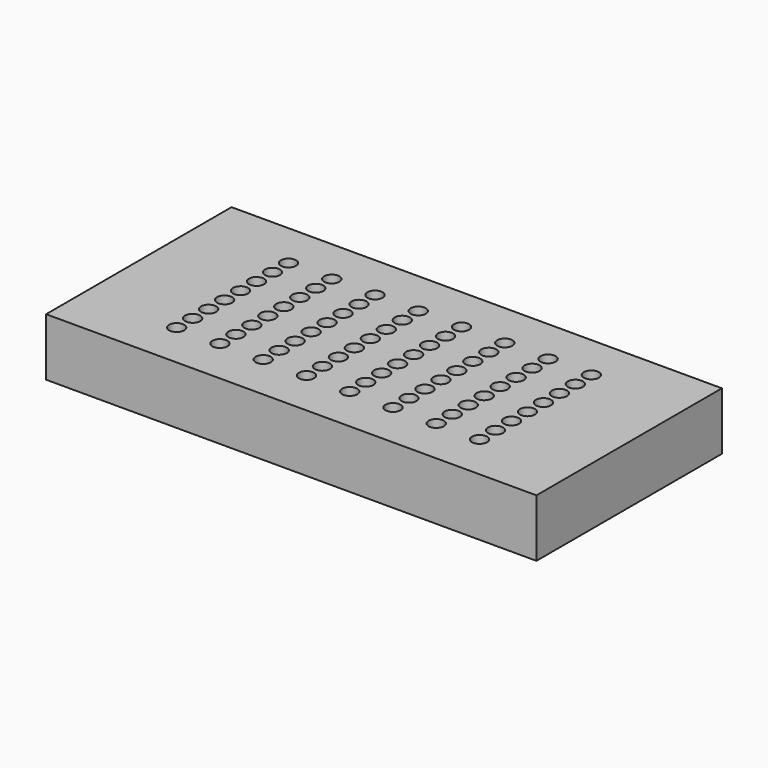
from build123d import *

# Parameters (mm, degrees)
F0_W     = 48
F0_H     = 22.15
F1_DEPTH = 4.98
F2_W     = 68
F2_H     = 32.15
F2_W_2   = 48
F2_H_2   = 22.15
F2_R     = 1.05
F3_DEPTH = 3
F4_DEPTH = 5


# Not quite as in the source:
# - a feature names something its author has since deleted; it is built from what else it names


with BuildPart() as f1:
    # F0 (on Top) → F1 (new body)
    with BuildSketch(Plane.XY):
        with Locations((-24, 11.075)):
            Rectangle(F0_W, F0_H)
    extrude(amount=F1_DEPTH)


with BuildPart() as f3:
    # F2 (on face) → F3 (new body)
    with BuildSketch(Plane.XY.offset(4.98)):
        with Locations((-24, 11.075)):
            Rectangle(F2_W, F2_H)
        with Locations((-24, 11.075)):
            Rectangle(F2_W_2, F2_H_2, mode=Mode.SUBTRACT)
        with Locations((-24, 11.075)):
            Rectangle(F2_W_2, F2_H_2)
        with Locations((-45, 1.384375)):
            Circle(F2_R, mode=Mode.SUBTRACT)
        with Locations((-39, 1.384375)):
            Circle(F2_R, mode=Mode.SUBTRACT)
        with Locations((-33, 1.384375)):
            Circle(F2_R, mode=Mode.SUBTRACT)
        with Locations((-27, 1.384375)):
            Circle(F2_R, mode=Mode.SUBTRACT)
        with Locations((-45, 4.153125)):
            Circle(F2_R, mode=Mode.SUBTRACT)
        with Locations((-45, 6.921875)):
            Circle(F2_R, mode=Mode.SUBTRACT)
        with Locations((-45, 9.690625)):
            Circle(F2_R, mode=Mode.SUBTRACT)
        with Locations((-39, 4.153125)):
            Circle(F2_R, mode=Mode.SUBTRACT)
        with Locations((-33, 4.153125)):
            Circle(F2_R, mode=Mode.SUBTRACT)
        with Locations((-39, 6.921875)):
            Circle(F2_R, mode=Mode.SUBTRACT)
        with Locations((-33, 6.921875)):
            Circle(F2_R, mode=Mode.SUBTRACT)
        with Locations((-27, 4.153125)):
            Circle(F2_R, mode=Mode.SUBTRACT)
        with Locations((-27, 6.921875)):
            Circle(F2_R, mode=Mode.SUBTRACT)
        with Locations((-39, 9.690625)):
            Circle(F2_R, mode=Mode.SUBTRACT)
        with Locations((-33, 9.690625)):
            Circle(F2_R, mode=Mode.SUBTRACT)
        with Locations((-27, 9.690625)):
            Circle(F2_R, mode=Mode.SUBTRACT)
        with Locations((-21, 1.384375)):
            Circle(F2_R, mode=Mode.SUBTRACT)
        with Locations((-15, 1.384375)):
            Circle(F2_R, mode=Mode.SUBTRACT)
        with Locations((-9, 1.384375)):
            Circle(F2_R, mode=Mode.SUBTRACT)
        with Locations((-3, 1.384375)):
            Circle(F2_R, mode=Mode.SUBTRACT)
        with Locations((-21, 4.153125)):
            Circle(F2_R, mode=Mode.SUBTRACT)
        with Locations((-21, 6.921875)):
            Circle(F2_R, mode=Mode.SUBTRACT)
        with Locations((-15, 4.153125)):
            Circle(F2_R, mode=Mode.SUBTRACT)
        with Locations((-9, 4.153125)):
            Circle(F2_R, mode=Mode.SUBTRACT)
        with Locations((-15, 6.921875)):
            Circle(F2_R, mode=Mode.SUBTRACT)
        with Locations((-9, 6.921875)):
            Circle(F2_R, mode=Mode.SUBTRACT)
        with Locations((-21, 9.690625)):
            Circle(F2_R, mode=Mode.SUBTRACT)
        with Locations((-15, 9.690625)):
            Circle(F2_R, mode=Mode.SUBTRACT)
        with Locations((-9, 9.690625)):
            Circle(F2_R, mode=Mode.SUBTRACT)
        with Locations((-3, 4.153125)):
            Circle(F2_R, mode=Mode.SUBTRACT)
        with Locations((-3, 6.921875)):
            Circle(F2_R, mode=Mode.SUBTRACT)
        with Locations((-3, 9.690625)):
            Circle(F2_R, mode=Mode.SUBTRACT)
        with Locations((-45, 12.459375)):
            Circle(F2_R, mode=Mode.SUBTRACT)
        with Locations((-45, 15.228125)):
            Circle(F2_R, mode=Mode.SUBTRACT)
        with Locations((-45, 17.996875)):
            Circle(F2_R, mode=Mode.SUBTRACT)
        with Locations((-39, 12.459375)):
            Circle(F2_R, mode=Mode.SUBTRACT)
        with Locations((-33, 12.459375)):
            Circle(F2_R, mode=Mode.SUBTRACT)
        with Locations((-27, 12.459375)):
            Circle(F2_R, mode=Mode.SUBTRACT)
        with Locations((-39, 15.228125)):
            Circle(F2_R, mode=Mode.SUBTRACT)
        with Locations((-33, 15.228125)):
            Circle(F2_R, mode=Mode.SUBTRACT)
        with Locations((-39, 17.996875)):
            Circle(F2_R, mode=Mode.SUBTRACT)
        with Locations((-33, 17.996875)):
            Circle(F2_R, mode=Mode.SUBTRACT)
        with Locations((-27, 15.228125)):
            Circle(F2_R, mode=Mode.SUBTRACT)
        with Locations((-27, 17.996875)):
            Circle(F2_R, mode=Mode.SUBTRACT)
        with Locations((-45, 20.765625)):
            Circle(F2_R, mode=Mode.SUBTRACT)
        with Locations((-39, 20.765625)):
            Circle(F2_R, mode=Mode.SUBTRACT)
        with Locations((-33, 20.765625)):
            Circle(F2_R, mode=Mode.SUBTRACT)
        with Locations((-27, 20.765625)):
            Circle(F2_R, mode=Mode.SUBTRACT)
        with Locations((-21, 12.459375)):
            Circle(F2_R, mode=Mode.SUBTRACT)
        with Locations((-15, 12.459375)):
            Circle(F2_R, mode=Mode.SUBTRACT)
        with Locations((-9, 12.459375)):
            Circle(F2_R, mode=Mode.SUBTRACT)
        with Locations((-21, 15.228125)):
            Circle(F2_R, mode=Mode.SUBTRACT)
        with Locations((-21, 17.996875)):
            Circle(F2_R, mode=Mode.SUBTRACT)
        with Locations((-15, 15.228125)):
            Circle(F2_R, mode=Mode.SUBTRACT)
        with Locations((-9, 15.228125)):
            Circle(F2_R, mode=Mode.SUBTRACT)
        with Locations((-15, 17.996875)):
            Circle(F2_R, mode=Mode.SUBTRACT)
        with Locations((-9, 17.996875)):
            Circle(F2_R, mode=Mode.SUBTRACT)
        with Locations((-3, 12.459375)):
            Circle(F2_R, mode=Mode.SUBTRACT)
        with Locations((-3, 15.228125)):
            Circle(F2_R, mode=Mode.SUBTRACT)
        with Locations((-3, 17.996875)):
            Circle(F2_R, mode=Mode.SUBTRACT)
        with Locations((-21, 20.765625)):
            Circle(F2_R, mode=Mode.SUBTRACT)
        with Locations((-15, 20.765625)):
            Circle(F2_R, mode=Mode.SUBTRACT)
        with Locations((-9, 20.765625)):
            Circle(F2_R, mode=Mode.SUBTRACT)
        with Locations((-3, 20.765625)):
            Circle(F2_R, mode=Mode.SUBTRACT)
    extrude(amount=F3_DEPTH)

    # F2 (on face) → F4 (join)
    with BuildSketch(Plane.XY.offset(4.98)):
        with Locations((-24, 11.075)):
            Rectangle(F2_W, F2_H)
        with Locations((-24, 11.075)):
            Rectangle(F2_W_2, F2_H_2, mode=Mode.SUBTRACT)
    extrude(amount=-F4_DEPTH)


solid = Compound([f1.part, f3.part])
